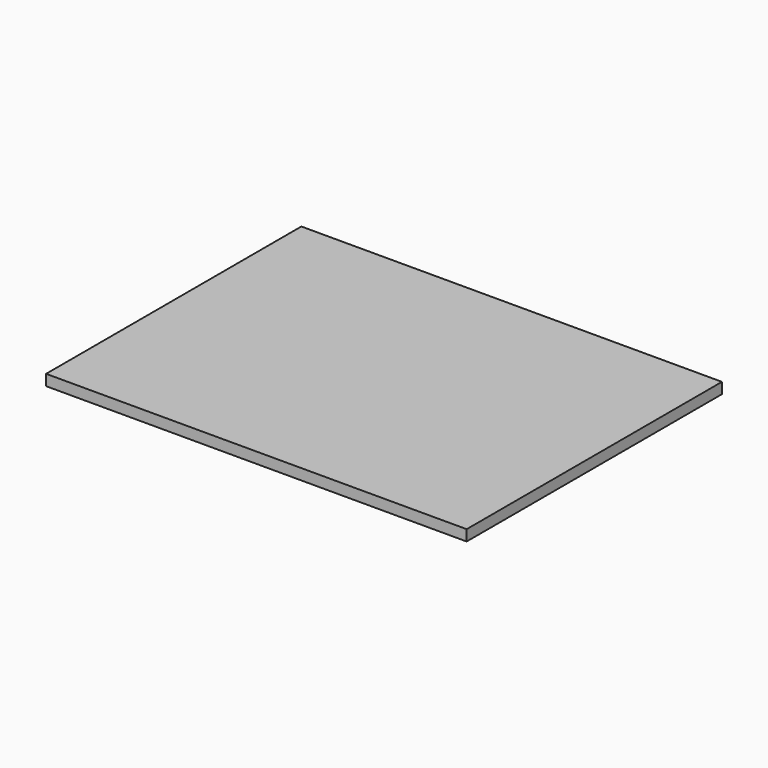
from build123d import *

# Parameters (mm, degrees)
F1_W     = 736.6
F1_H     = 558.8
F2_DEPTH = 19.05


# Not quite as in the source:
# - a feature of the source that left no trace in its solid (it failed there, or was rolled back) is left out


with BuildPart() as f2:
    # F1 (on offset) → F2 (new body)
    with BuildSketch(Plane.XY.offset(711.2)):
        Rectangle(F1_W, F1_H)
    extrude(amount=-F2_DEPTH)


solid = f2.part
